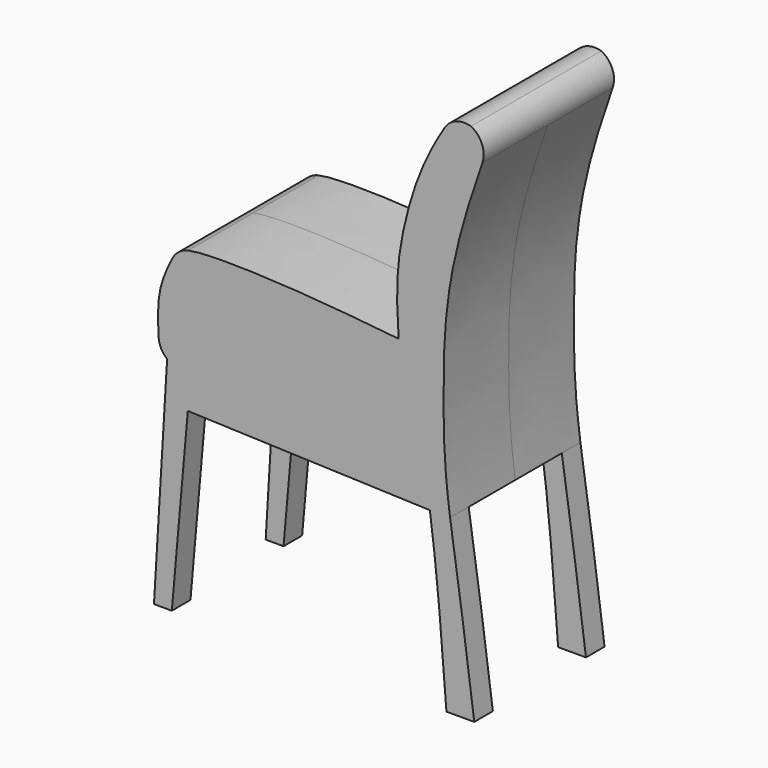
from build123d import *

# Parameters (mm, degrees)
F1_DEPTH    = 17.78
F2_DEPTH    = 5.08
F3_T1_DEPTH = 35.8062984981
F3_T3_DEPTH = 30.4788212018
F3_T5_DEPTH = 42.8132024584
F3_T7_DEPTH = 47.9220802156


# Not quite as in the source:
# - a fillet or chamfer that OpenCascade refuses, or shapes differently, is made with other operations: its cross-section is extruded or revolved along the edge and cut away or added


with BuildPart() as f1:
    # F0 (on Front) → F1 (new body)
    with BuildSketch(Plane.XZ):
        with BuildLine():
            add(Edge.make_bspline(
                [(-37.0363406837, 14.0804359689), (-35.9072652533, 14.4664877028), (-32.2858897401, 15.7047028462), (-9.9762911381, 14.9349511241), (4.1730021841, 13.4876905203), (11.3340960816, 12.755217962)],
                knots=[0, 0, 0, 0, 0.1828362337, 0.5864255319, 1, 1, 1, 1], degree=3))
            add(Edge.make_bspline(
                [(-40.7805715998, -7.587400265), (-41.1571131004, -3.1737627482), (-41.8654052574, 5.1284956529), (-38.5767054854, 11.224964985), (-37.0363406837, 14.0804359689)],
                knots=[0, 0, 0, 0, 0.5316189046, 1, 1, 1, 1], degree=3))
            add(Edge.make_bspline(
                [(-39.2111837864, -7.587400265), (-39.7343130575, -7.587400265), (-40.2574423287, -7.587400265), (-40.7805715998, -7.587400265)],
                knots=[0, 0, 0, 0, 1.5693878134, 1.5693878134, 1.5693878134, 1.5693878134], degree=3))
            add(Edge.make_bspline(
                [(-39.7181957521, -16.0697158426), (-39.5491917635, -13.2422773167), (-39.380187775, -10.4148387909), (-39.2111837864, -7.587400265)],
                knots=[39.5947721886, 39.5947721886, 39.5947721886, 39.5947721886, 48.0922270247, 48.0922270247, 48.0922270247, 48.0922270247], degree=3))
            Line((-39.7181957521, -16.0697158426), (-34.6953757107, -16.0697158426))
            add(Edge.make_bspline(
                [(18.1377418348, -17.9571639745), (1.0042935619, -17.3535464951), (-17.5619274378, -16.673333322), (-34.6953757107, -16.0697158426)],
                knots=[0, 0, 0, 0, 52.8668210698, 52.8668210698, 52.8668210698, 52.8668210698], degree=3))
            Line((18.1377418348, -17.9571639745), (22.5548642091, -17.9571639745))
            add(Edge.make_bspline(
                [(31.0414787382, 56.6072203219), (29.451074184, 52.0886125693), (26.2723609904, 43.0573519115), (22.6536296154, 29.3346938321), (21.2600863367, 16.9929663306), (21.1386219291, 7.653611923), (21.0411584125, -5.3538743468), (22.1296230711, -14.7801385495), (22.5548642091, -17.9571639745)],
                knots=[0, 0, 0, 0, 0.1361460961, 0.2721127721, 0.3967558164, 0.5055490646, 0.651139282, 0.7233224297, 0.7233224297, 0.7233224297, 0.7233224297], degree=3))
            add(Edge.make_bspline(
                [(22.9297485203, 59.1378286481), (23.9176047114, 59.2712834835), (26.2358281174, 59.584464821), (29.2892185653, 57.692797983), (31.0414787382, 56.6072203219)],
                knots=[0, 0, 0, 0, 0.4261263986, 1, 1, 1, 1], degree=3))
            add(Edge.make_bspline(
                [(11.3340960816, 12.755217962), (11.0324387543, 17.4888695508), (10.3827239426, 27.6842908865), (15.5238608305, 47.2129566198), (20.6106760328, 55.4036857883), (22.9297485203, 59.1378286481)],
                knots=[0, 0, 0, 0, 0.3204519046, 0.6901949001, 1, 1, 1, 1], degree=3))
        make_face()
    extrude(amount=F1_DEPTH)

    # F0 (on Front) → F2 (join)
    with BuildSketch(Plane.XZ):
        with BuildLine():
            Line((-34.6953757107, -16.0697158426), (-39.7181957521, -16.0697158426))
            add(Edge.make_bspline(
                [(-42.0806705952, -55.593945086), (-41.2931789808, -42.4192020049), (-40.5056873665, -29.2444589237), (-39.7181957521, -16.0697158426)],
                knots=[0, 0, 0, 0, 39.5947721886, 39.5947721886, 39.5947721886, 39.5947721886], degree=3))
            add(Edge.make_bspline(
                [(-38.1803736091, -55.593945086), (-39.4804726044, -55.593945086), (-40.7805715998, -55.593945086), (-42.0806705952, -55.593945086)],
                knots=[0, 0, 0, 0, 3.9002969861, 3.9002969861, 3.9002969861, 3.9002969861], degree=3))
            add(Edge.make_bspline(
                [(-34.6953757107, -16.0697158426), (-35.8570416768, -29.2444589237), (-37.018707643, -42.4192020049), (-38.1803736091, -55.593945086)],
                knots=[0, 0, 0, 0, 39.6775743668, 39.6775743668, 39.6775743668, 39.6775743668], degree=3))
        make_face()
        with BuildLine():
            add(Edge.make_bspline(
                [(22.5548642091, -17.9571639745), (23.1406834486, -22.3338868554), (25.110997642, -34.7891360369), (26.7680646459, -47.4091949068), (27.8295651078, -55.4934777319)],
                knots=[0.7233224297, 0.7233224297, 0.7233224297, 0.7233224297, 0.8227631303, 1, 1, 1, 1], degree=3))
            Line((22.5548642091, -17.9571639745), (18.1377418348, -17.9571639745))
            add(Edge.make_bspline(
                [(21.7594448477, -55.4934777319), (21.0663466567, -46.5798409174), (19.8733367549, -31.2370552726), (18.6502547708, -21.8786527932), (18.1377418348, -17.9571639745)],
                knots=[0, 0, 0, 0, 0.5809660006, 1, 1, 1, 1], degree=3))
            add(Edge.make_bspline(
                [(27.8295651078, -55.4934777319), (25.8061916878, -55.4934777319), (23.7828182677, -55.4934777319), (21.7594448477, -55.4934777319)],
                knots=[0, 0, 0, 0, 6.0701202601, 6.0701202601, 6.0701202601, 6.0701202601], degree=3))
        make_face()
    extrude(amount=F2_DEPTH)

    # F3: fillet of radius 5.08 on 4 edges, made by hand

    # F3_s2 → F3_t1 (cut)
    with BuildSketch(Plane.XZ.offset(-9.0131492491)):
        with BuildLine():
            ThreePointArc((-41.0654329019, -3.9934120152), (-40.5113634996, -5.9828767727), (-39.2111837864, -7.587400265))
            Line((-39.2111837864, -7.587400265), (-39.2754713457, -7.666074719))
            ThreePointArc((-39.2754713457, -7.666074719), (-39.9958776931, -7.689000265), (-40.7805715998, -7.689000265))
            Line((-40.7805715998, -7.689000265), (-40.8818038663, -7.5960367127))
            ThreePointArc((-40.8818038663, -7.5960367127), (-41.0323979759, -5.7992458414), (-41.1668054436, -4.0002067042))
            Line((-41.1668054436, -4.0002067042), (-41.0654329019, -3.9934120152))
        make_face()
    extrude(amount=F3_T1_DEPTH, mode=Mode.SUBTRACT)

    # F3_s4 → F3_t3 (cut)
    with BuildSketch(Plane.XZ.offset(-6.3494106009)):
        with BuildLine():
            ThreePointArc((-34.5963046101, 14.7851531861), (-36.6248709598, 13.860065118), (-38.061951969, 12.1554632461))
            Line((-38.061951969, 12.1554632461), (-38.1521078254, 12.2023085399))
            ThreePointArc((-38.1521078254, 12.2023085399), (-37.6424780921, 13.1678308874), (-37.1257598745, 14.1286725558))
            Line((-37.1257598745, 14.1286725558), (-37.0692112747, 14.1765717284))
            ThreePointArc((-37.0692112747, 14.1765717284), (-35.8572472499, 14.5711412658), (-34.6171475194, 14.8845922787))
            Line((-34.6171475194, 14.8845922787), (-34.5963046101, 14.7851531861))
        make_face()
    extrude(amount=F3_T3_DEPTH, mode=Mode.SUBTRACT)

    # F3_s6 → F3_t5 (cut)
    with BuildSketch(Plane.XZ.offset(-12.5166012292)):
        with BuildLine():
            ThreePointArc((27.8862106757, 58.4307700125), (24.2228232961, 58.7447859797), (21.3071174751, 56.5047697552))
            Line((21.3071174751, 56.5047697552), (21.220258421, 56.5574771049))
            ThreePointArc((21.220258421, 56.5574771049), (22.0285709469, 57.8767827762), (22.8434388423, 59.1914308821))
            Line((22.8434388423, 59.1914308821), (22.9161463902, 59.2385140098))
            ThreePointArc((22.9161463902, 59.2385140098), (25.4817069799, 59.3415947788), (27.9309334856, 58.5219973674))
            Line((27.9309334856, 58.5219973674), (27.8862106757, 58.4307700125))
        make_face()
    extrude(amount=F3_T5_DEPTH, mode=Mode.SUBTRACT)

    # F3_s8 → F3_t7 (cut)
    with BuildSketch(Plane.XZ.offset(-15.0710401078)):
        with BuildLine():
            ThreePointArc((29.6134478053, 52.5339448765), (29.1735899714, 56.8129265835), (25.6089175294, 59.2204709225))
            Line((25.6089175294, 59.2204709225), (25.6247878066, 59.3208237715))
            ThreePointArc((25.6247878066, 59.3208237715), (28.4954140197, 58.2321967662), (31.0949864807, 56.6935886118))
            Line((31.0949864807, 56.6935886118), (31.1373157967, 56.5734887606))
            ThreePointArc((31.1373157967, 56.5734887606), (30.4214522449, 54.5375989985), (29.709408688, 52.5005672046))
            Line((29.709408688, 52.5005672046), (29.6134478053, 52.5339448765))
        make_face()
    extrude(amount=F3_T7_DEPTH, mode=Mode.SUBTRACT)

    # F5: F1 across plane


with BuildPart() as f1_1:
    add(f1.part)
    add(f1.part.mirror(Plane(origin=(-3.442122023, -17.78, 6.1004007624), x_dir=(1, 0, 0), z_dir=(0, -1, 0))))


solid = f1_1.part
